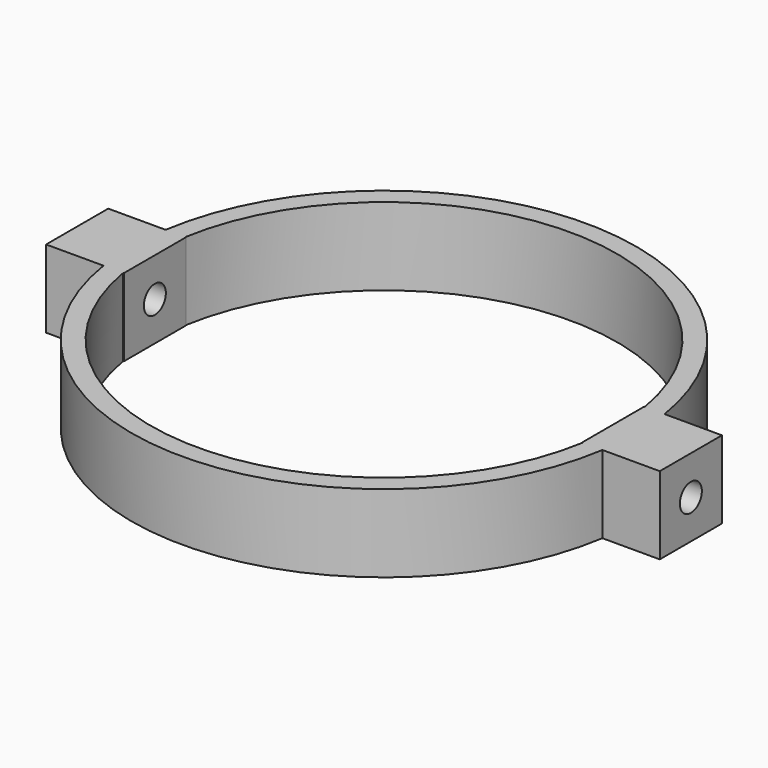
from build123d import *

# Parameters (mm, degrees)
F0_R     = 41.275
F0_R_2   = 38.1
F1_DEPTH = 12.7
F3_W     = 12.7
F3_H     = 12.7
F4_DEPTH = 12.7
F6_W     = 12.7
F6_H     = 12.7
F7_DEPTH = 12.7
F9_D     = 4.4958


with BuildPart() as f1:
    # F0 (on Top) → F1 (new body)
    with BuildSketch(Plane.XY):
        Circle(F0_R)
        Circle(F0_R_2, mode=Mode.SUBTRACT)
    extrude(amount=F1_DEPTH)

    # F3 (on offset) → F4 (join)
    with BuildSketch(Plane.YZ.offset(37.465)):
        with Locations((0, 6.35)):
            Rectangle(F3_W, F3_H)
    extrude(amount=F4_DEPTH)

    # F6 (on offset) → F7 (join)
    with BuildSketch(Plane.YZ.offset(-37.465)):
        with Locations((0, 6.35)):
            Rectangle(F6_W, F6_H)
    extrude(amount=-F7_DEPTH)

    # F9 (through all)
    with Locations(Plane(origin=(-50.165, 0, 0), x_dir=(0, -1, 0), z_dir=(-1, 0, 0))):
        with Locations((0, 6.35)):
            Hole(F9_D / 2)


solid = f1.part
